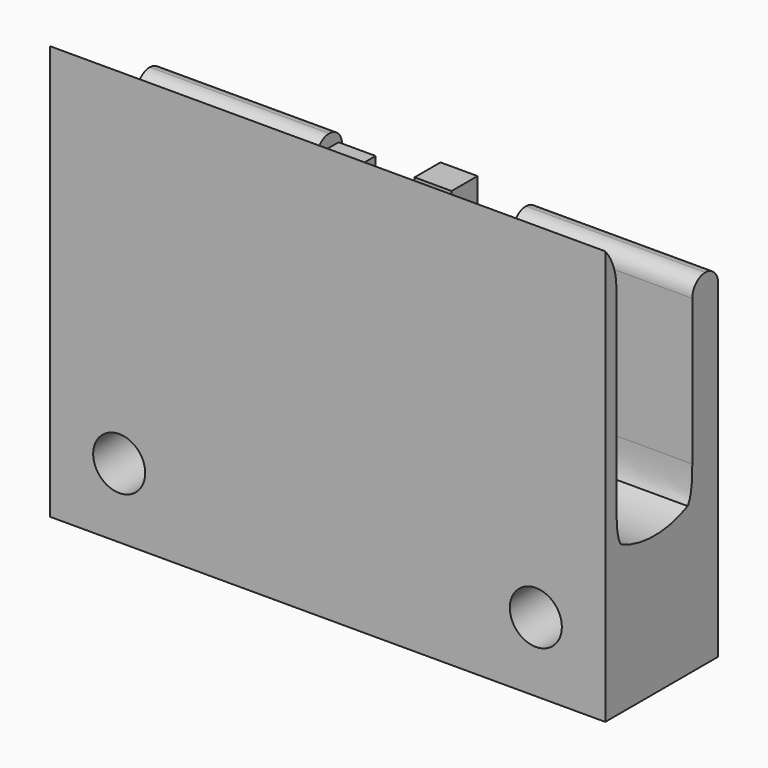
from build123d import *

# Parameters (mm, degrees)
F1_DEPTH        = 3.2
F2_DEPTH        = 24
F4_DEPTH        = 35.8010001
F5_W            = 17
F5_H            = 13.8
F6_DEPTH        = 2.8
F7_R            = 1.39999
F8_T1_DEPTH     = 64.2480768093
F9_R            = 2
F10_D           = 4.4958
F10_CSINK_D     = 9.1186
F10_CSINK_ANGLE = 82


# Not quite as in the source:
# - a fillet or chamfer that OpenCascade refuses, or shapes differently, is made with other operations: its cross-section is extruded or revolved along the edge and cut away or added
# - a fillet or chamfer is up to 0.001 mm smaller than in the source, because OpenCascade refuses the exact size


with BuildPart() as f1:
    # F0 (on Right) → F1 (new body)
    with BuildSketch(Plane.YZ):
        with BuildLine():
            Line((1.2, 15.8), (1.2, 35.8))
            Line((1.2, 35.8), (0, 35.8))
            Line((0, 35.8), (0, 0))
            Line((0, 0), (12.2, 0))
            Line((12.2, 0), (12.2, 29.8))
            Line((12.2, 29.8), (9.4, 29.8))
            Line((9.4, 29.8), (9.4, 15.8))
            add(Edge.make_bspline(
                [(9.4, 15.8), (9.4, 13.7632392675), (9.1505151562, 13.2120574221), (8.9, 12.8)],
                knots=[0, 0, 0, 0, 3.0413812651, 3.0413812651, 3.0413812651, 3.0413812651], degree=3))
            ThreePointArc((8.9, 12.8), (5.3, 12), (1.7, 12.8))
            add(Edge.make_bspline(
                [(1.2, 15.8), (1.2, 13.7632392675), (1.4494848438, 13.2120574221), (1.7, 12.8)],
                knots=[0, 0, 0, 0, 3.0413812651, 3.0413812651, 3.0413812651, 3.0413812651], degree=3))
        make_face()
    extrude(amount=F1_DEPTH)


with BuildPart() as f2:
    # F0 (on Right) → F2 (new body, symmetric)
    with BuildSketch(Plane.YZ):
        with BuildLine():
            Line((1.2, 15.8), (1.2, 35.8))
            Line((1.2, 35.8), (0, 35.8))
            Line((0, 35.8), (0, 0))
            Line((0, 0), (12.2, 0))
            Line((12.2, 0), (12.2, 29.8))
            Line((12.2, 29.8), (9.4, 29.8))
            Line((9.4, 29.8), (9.4, 15.8))
            add(Edge.make_bspline(
                [(9.4, 15.8), (9.4, 13.7632392675), (9.1505151562, 13.2120574221), (8.9, 12.8)],
                knots=[0, 0, 0, 0, 3.0413812651, 3.0413812651, 3.0413812651, 3.0413812651], degree=3))
            ThreePointArc((8.9, 12.8), (5.3, 12), (1.7, 12.8))
            add(Edge.make_bspline(
                [(1.2, 15.8), (1.2, 13.7632392675), (1.4494848438, 13.2120574221), (1.7, 12.8)],
                knots=[0, 0, 0, 0, 3.0413812651, 3.0413812651, 3.0413812651, 3.0413812651], degree=3))
        make_face()
    extrude(amount=F2_DEPTH, both=True)

    # F3 (on Top) → F4 (cut, through all)
    with BuildSketch(Plane.XY):
        with BuildLine():
            Line((1.85, 8.2), (-1.85, 8.2))
            ThreePointArc((-1.85, 8.2), (-5.25, 4.8), (-1.85, 1.4))
            Line((-1.85, 1.4), (1.85, 1.4))
            ThreePointArc((1.85, 1.4), (5.25, 4.8), (1.85, 8.2))
        make_face()
    extrude(amount=F4_DEPTH, mode=Mode.SUBTRACT)

    # F5 (on face) → F6 (cut, through all)
    with BuildSketch(Plane(origin=(0, 12.2, 0), x_dir=(-1, 0, 0), z_dir=(0, 1, 0))):
        with Locations((0, 22.9)):
            Rectangle(F5_W, F5_H)
    extrude(amount=-F6_DEPTH, mode=Mode.SUBTRACT)

    # F7 (radius 1.4 in the source; OpenCascade refuses exactly that, so slightly less here)
    f7_edges = [f2.edges().sort_by_distance(p)[0] for p in [
        (16.25, 12.2, 29.8),
        (-16.25, 12.2, 29.8),
        (-16.25, 9.4, 29.8),
        (16.25, 9.4, 29.8),
    ]]
    fillet(f7_edges, radius=F7_R)

    # F8: fillet of radius 5 on 1 edges, made by hand

    # F8_s2 → F8_t1 (cut)
    with BuildSketch(Plane.YZ.offset(-32.1240384046)):
        with BuildLine():
            ThreePointArc((0, 35.8), (0.8904157598, 34.2824354457), (1.2, 32.5503846381))
            Line((1.2, 32.5503846381), (1.2, 35.8))
            Line((1.2, 35.8), (0, 35.8))
        make_face()
    extrude(amount=F8_T1_DEPTH, mode=Mode.SUBTRACT)

    # F9
    f9_edges = [f2.edges().sort_by_distance(p)[0] for p in [
        (8.5, 10.8, 16),
        (-8.5, 10.8, 16),
    ]]
    fillet(f9_edges, radius=F9_R)

    # F10 (through all)
    with Locations(Plane(origin=(0, 12.2, 0), x_dir=(-1, 0, 0), z_dir=(0, 1, 0))):
        with Locations((-18, 6), (18, 6)):
            CounterSinkHole(F10_D / 2, F10_CSINK_D / 2, counter_sink_angle=F10_CSINK_ANGLE)


solid = Compound([f1.part, f2.part])
